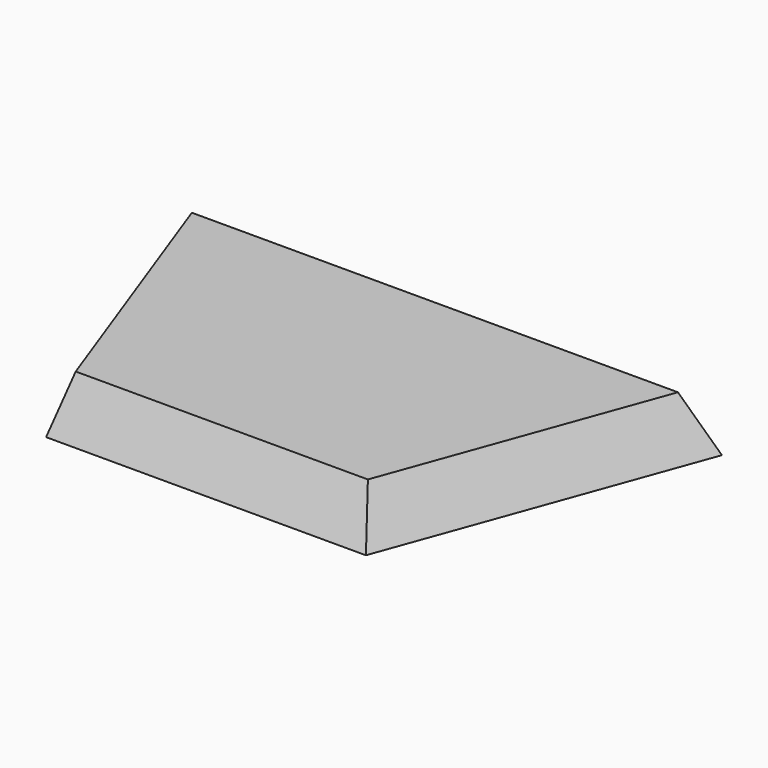
from build123d import *

# Parameters (mm, degrees)
F1_DEPTH = 6.35
F1_TAPER = 20


with BuildPart() as f1:
    # F0 (on Top) → F1 (new body)
    with BuildSketch(Plane.XY):
        Polygon((31.261141, 24.280021), (-32.238859, 24.280021), (-19.207891, -11.522268), (18.230174, -11.522268), align=None)
    extrude(amount=F1_DEPTH, taper=F1_TAPER)


solid = f1.part
